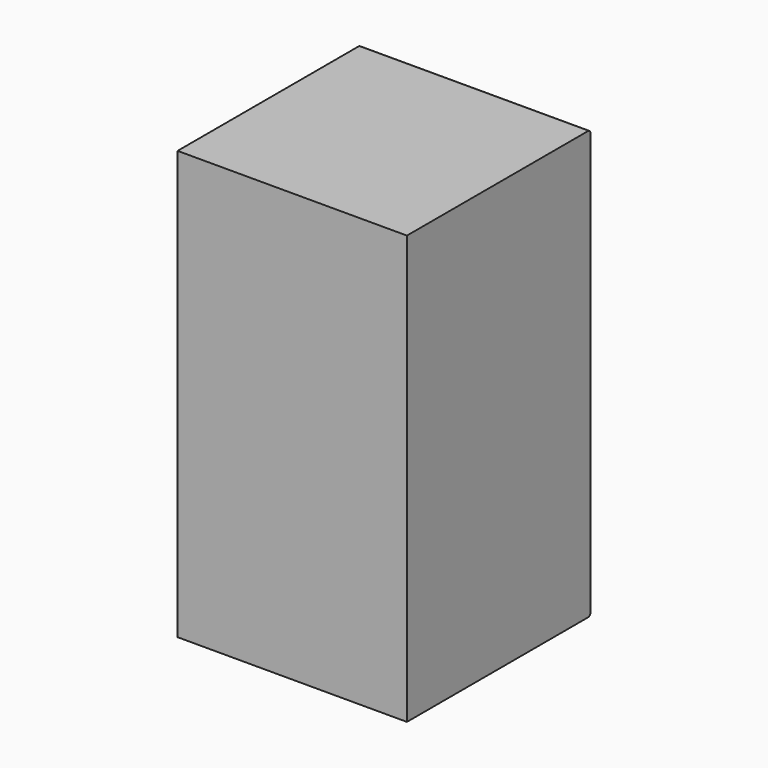
from build123d import *

# Parameters (mm, degrees)
F0_W     = 381
F0_H     = 711.2
F1_DEPTH = 190.5
F2_T     = -6.35
F4_W     = 374.65
F4_H     = 698.5
F4_W_2   = 216.2134721875
F4_H_2   = 11.9601786137
F4_H_3   = 12.0113417506
F4_H_4   = 13.8943791389
F4_H_5   = 13.2367163897
F5_DEPTH = 6.35
F6_R     = 5.08
F8_DEPTH = 6.35


# Not quite as in the source:
# - a feature names something its author has since deleted; it is built from what else it names


with BuildPart() as f1:
    # F0 (on Front) → F1 (new body, symmetric)
    with BuildSketch(Plane.XZ):
        with Locations((-19.8015896951, 73.5329994828)):
            Rectangle(F0_W, F0_H)
    extrude(amount=F1_DEPTH, both=True)

    # F2
    f2_openings = [f1.faces().sort_by_distance(p)[0] for p in [
        (-19.80159, 190.5, 73.532999),
    ]]
    offset(amount=F2_T, openings=f2_openings)

    # F4 (on offset) → F5 (join, symmetric)
    with BuildSketch(Plane(origin=(0, 184.15, 0), x_dir=(-1, 0, 0), z_dir=(0, 1, 0))):
        with Locations((18.9778648138, 74.4046084881)):
            Rectangle(F4_W, F4_H)
        Polygon((-88.1409570575, 335.4734778404), (-88.1409570575, 348.0727672577), (128.07251513, 348.0727672577), (128.07251513, 335.4734778404), (128.07251513, 323.5132992268), (128.07251513, 309.8019063473), (128.07251513, 297.7905645967), (128.07251513, 286.5811288357), (128.07251513, 272.6867496967), (128.07251513, 260.7450783253), (128.07251513, 247.5083619356), (-88.1409570575, 247.5083619356), (-88.1409570575, 260.7450783253), (-88.1409570575, 272.6867496967), (-88.1409570575, 286.5811288357), (-88.1409570575, 297.7905645967), (-88.1409570575, 309.8019063473), (-88.1409570575, 323.5132992268), align=None, mode=Mode.SUBTRACT)
        with Locations((19.9657790363, 329.4933885336)):
            Rectangle(F4_W_2, F4_H_2)
        with Locations((19.9657790363, 303.796235472)):
            Rectangle(F4_W_2, F4_H_3)
        with Locations((19.9657790363, 279.6339392662)):
            Rectangle(F4_W_2, F4_H_4)
        with Locations((19.9657790363, 254.1267201304)):
            Rectangle(F4_W_2, F4_H_5)
    extrude(amount=F5_DEPTH, both=True)

    # F6
    f6_edges = [f1.edges().sort_by_distance(p)[0] for p in [
        (-19.80159, 190.5, 429.132999),
        (-19.80159, 190.5, -282.067001),
    ]]
    fillet(f6_edges, radius=F6_R)

    # F7 (on face) → F8 (cut)
    with BuildSketch(Plane(origin=(0, 190.5, 0), x_dir=(-1, 0, 0), z_dir=(0, 1, 0))):
        with BuildLine():
            ThreePointArc((-123.7823893566, 49.7743694082), (-128.773401113, 46.0705343361), (-130.1186089124, 40.0026674482))
            Line((-130.1186089124, 40.0026674482), (-108.4877372412, -114.6825799083))
            ThreePointArc((-108.4877372412, -114.6825799083), (-105.5180801987, -120.1587572974), (-99.6834033498, -122.3413996903))
            Line((-99.6834033498, -122.3413996903), (-8.89, -122.3413996903))
            ThreePointArc((-8.89, -122.3413996903), (-2.6038207153, -119.7375789751), (0, -113.4513996903))
            Line((0, -113.4513996903), (0, 73.7231935432))
            ThreePointArc((0, 73.7231935432), (-3.5472215301, 80.8286012177), (-11.3581143356, 82.2637152852))
            Line((-11.3581143356, 82.2637152852), (-123.7823893566, 49.7743694082))
        make_face()
    extrude(amount=-F8_DEPTH, mode=Mode.SUBTRACT)


solid = f1.part
